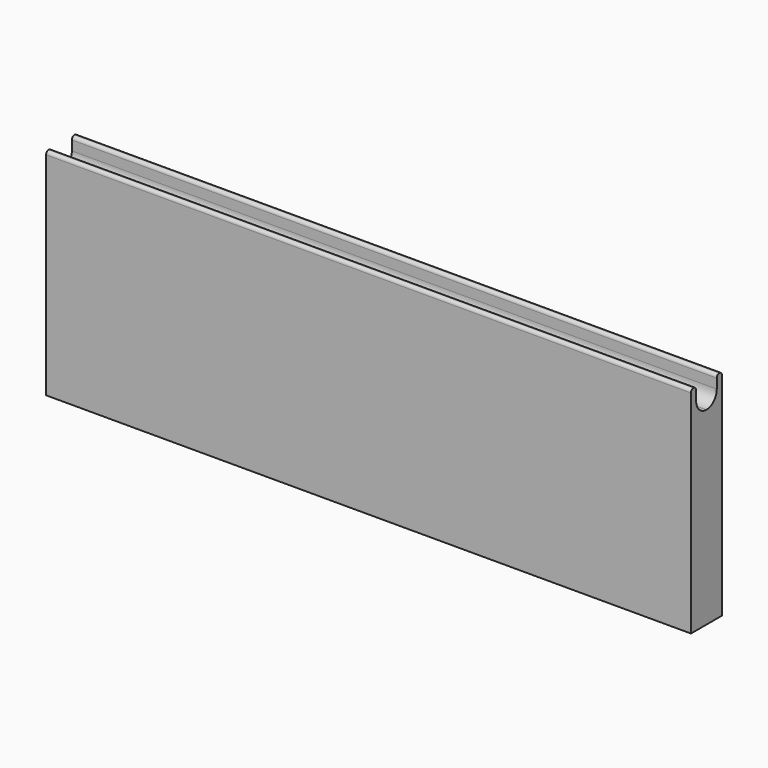
from build123d import *

# Parameters (mm, degrees)
F0_W     = 300
F0_H     = 100
F1_DEPTH = 9
F2_W     = 12
F2_H     = 12
F3_DEPTH = 300.001
F4_R     = 5.99999
F5_R     = 1.49999


# Not quite as in the source:
# - a fillet or chamfer is up to 0.001 mm smaller than in the source, because OpenCascade refuses the exact size


with BuildPart() as f1:
    # F0 (on Front) → F1 (new body, symmetric)
    with BuildSketch(Plane.XZ):
        with Locations((-3.7248600274, -105.7776198197)):
            Rectangle(F0_W, F0_H)
    extrude(amount=F1_DEPTH, both=True)

    # F2 (on face) → F3 (cut, through all)
    with BuildSketch(Plane.YZ.offset(146.2751399726)):
        with Locations((0, -61.7776198197)):
            Rectangle(F2_W, F2_H)
    extrude(amount=-F3_DEPTH, mode=Mode.SUBTRACT)

    # F4 (radius 6 in the source; OpenCascade refuses exactly that, so slightly less here)
    f4_edges = [f1.edges().sort_by_distance(p)[0] for p in [
        (-3.72486, 6, -67.77762),
        (-3.72486, -6, -67.77762),
    ]]
    fillet(f4_edges, radius=F4_R)

    # F5 (radius 1.5 in the source; OpenCascade refuses exactly that, so slightly less here)
    f5_edges = [f1.edges().sort_by_distance(p)[0] for p in [
        (-3.72486, -9, -55.77762),
        (-3.72486, -6, -55.77762),
        (-3.72486, 6, -55.77762),
        (-3.72486, 9, -55.77762),
    ]]
    fillet(f5_edges, radius=F5_R)


solid = f1.part
